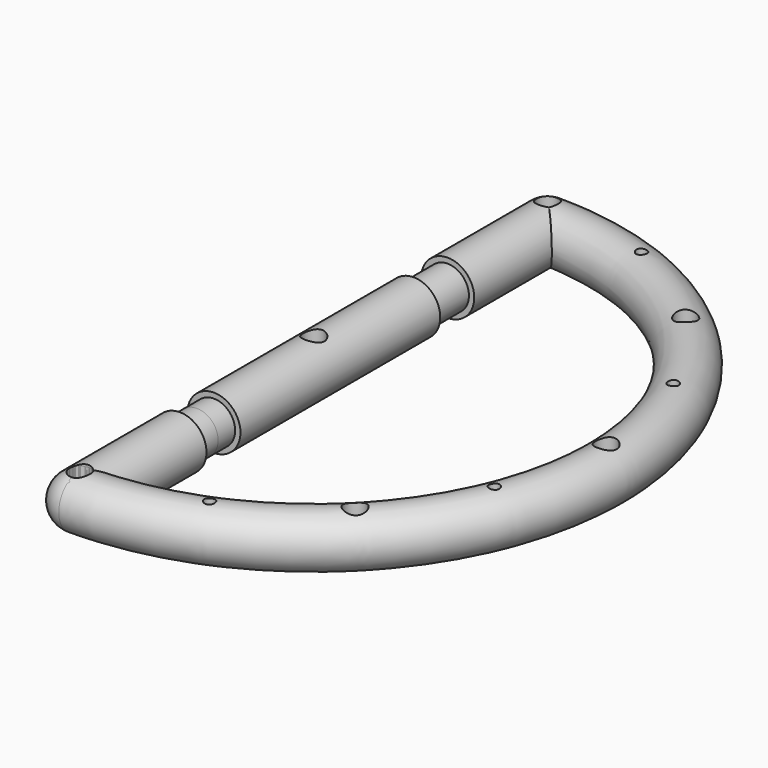
from build123d import *

# Parameters (mm, degrees)
F4_R           = 5
F6_DEPTH       = 110
F8_R           = 5
F12_R          = 2
F13_DEPTH      = 25
F13_DEPTH_BACK = 3
F14_R          = 1
F15_DEPTH      = 5.0010001003
F15_DEPTH_BACK = 5.0010001
F16_R          = 5
F16_R_2        = 4
F17_R          = 5
F17_R_2        = 4
F18_DEPTH      = 4


with BuildPart() as f6:
    # F4 (on Front) → F6 (new body)
    with BuildSketch(Plane.XZ):
        Circle(F4_R)
    extrude(amount=F6_DEPTH)

    # F9: sweep along a path in F7
    with BuildLine(Plane.XY) as f9_path:
        ThreePointArc((0, 0), (55, -55), (0, -110))
    # F8 (on Right) → F9 (sweep)
    with BuildSketch(Plane.YZ):
        with Locations((-110, 0)):
            Circle(F8_R)
    sweep(path=f9_path.line)

    # F6_face (on face) → F10 (revolve)
    with BuildSketch(Plane(origin=(-2.1220659079, 0, 0), x_dir=(1, 0, 0), z_dir=(0, 1, 0))):
        with BuildLine():
            Line((2.1220659079, -5), (2.1220659079, 5))
            ThreePointArc((2.1220659079, 5), (-2.8779340921, 0), (2.1220659079, -5))
        make_face()
    revolve(axis=Axis((0, 0, 0), (0, 0, 1)))


with BuildPart() as f11:
    # F9_face (on face) → F11 (revolve)
    with BuildSketch(Plane(origin=(0, -112.1220659079, 0), x_dir=(0, -1, 0), z_dir=(-1, 0, 0))):
        with BuildLine():
            Line((-2.1220659079, 5), (-2.1220659079, -5))
            ThreePointArc((-2.1220659079, -5), (2.8779340921, 0), (-2.1220659079, 5))
        make_face()
    revolve(axis=Axis((0, -110, 0), (0, 0, -1)))


with BuildPart() as f13_tool:
    # F12 (on Top) → F13 (new body, two sides)
    with BuildSketch(Plane.XY) as f13_sk:
        Circle(F12_R)
        with Locations((0, -110)):
            Circle(F12_R)
        with Locations((38.8908729653, -93.8908729653)):
            Circle(F12_R)
        with Locations((55, -55)):
            Circle(F12_R)
        with Locations((38.8908729653, -16.1091270347)):
            Circle(F12_R)
        with Locations((0, -55)):
            Circle(F12_R)
    extrude(amount=F13_DEPTH)
    extrude(f13_sk.sketch, amount=-F13_DEPTH_BACK)


with BuildPart() as f6_1:
    add(f6.part)

    # F13: cut by f13_tool
    add(f13_tool.part, mode=Mode.SUBTRACT)

    # F14 (on Top) → F15 (cut, two sides)
    with BuildSketch(Plane.XY) as f15_sk:
        with Locations((21.0475887801, -105.8133742881)):
            Circle(F14_R)
        with Locations((50.8133742881, -76.0475887801)):
            Circle(F14_R)
        with Locations((50.8133742881, -33.9524112199)):
            Circle(F14_R)
        with Locations((21.0475887801, -4.1866257119)):
            Circle(F14_R)
    extrude(amount=F15_DEPTH, mode=Mode.SUBTRACT)
    extrude(f15_sk.sketch, amount=-F15_DEPTH_BACK, mode=Mode.SUBTRACT)

    # F16 (on offset) + F17 (on offset) → F18 (cut, symmetric)
    with BuildSketch(Plane.XZ.offset(82.5)):
        Circle(F16_R)
        Circle(F16_R_2, mode=Mode.SUBTRACT)
    with BuildSketch(Plane.XZ.offset(27.5)):
        Circle(F17_R)
        Circle(F17_R_2, mode=Mode.SUBTRACT)
    extrude(amount=F18_DEPTH, both=True, mode=Mode.SUBTRACT)


with BuildPart() as f11_1:
    add(f11.part)

    # F13: cut by f13_tool
    add(f13_tool.part, mode=Mode.SUBTRACT)


solid = Compound([f6_1.part, f11_1.part])
